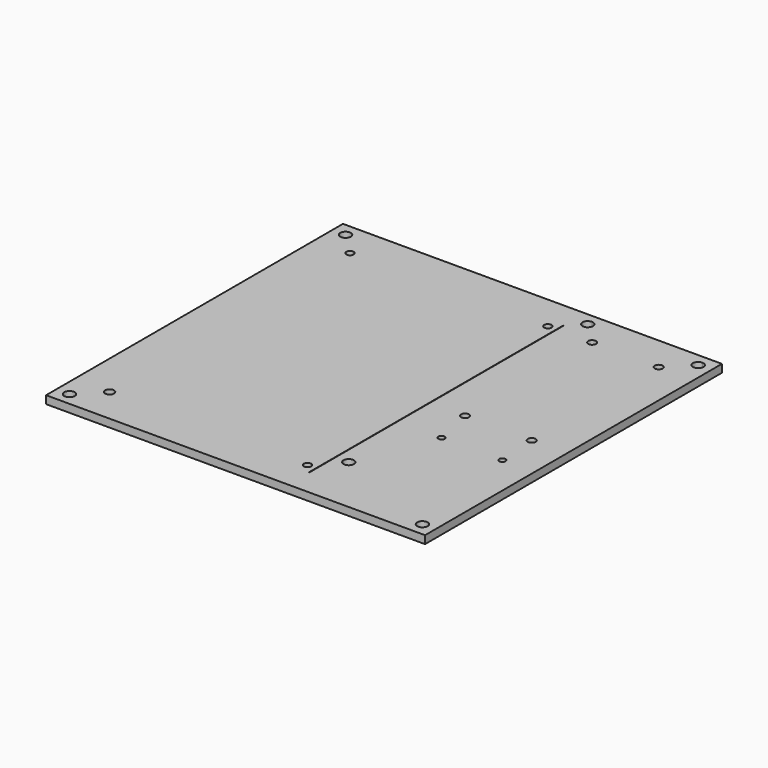
from build123d import *

# Parameters (mm, degrees)
F0_R     = 1.5
F0_W     = 3
F0_H     = 5
F0_W_2   = 4
F0_H_2   = 75.28
F0_H_3   = 40.64
F0_H_4   = 5.08
F1_DEPTH = 3


# Not quite as in the source:
# - a feature names something its author has since deleted; it is built from what else it names


with BuildPart() as f1:
    # F0 (on Top) → F1 (new body)
    with BuildSketch(Plane.XY):
        with BuildLine():
            Line((-134.3440142274, -1.256315279), (-139.3440142274, -1.256315279))
            Line((-139.3440142274, -1.256315279), (-139.3440142274, -6.256315279))
            Line((-139.3440142274, -6.256315279), (-136.3440142274, -6.256315279))
            ThreePointArc((-136.3440142274, -6.256315279), (-135.7582277898, -4.8421017166), (-134.3440142274, -4.256315279))
            Line((-134.3440142274, -4.256315279), (-134.3440142274, -1.256315279))
        make_face()
        Polygon((-139.3440142274, -6.256315279), (-139.3440142274, -1.256315279), (-221.3440142274, -1.256315279), (-221.3440142274, -6.256315279), (-221.3440142274, -11.256315279), (-217.9440142274, -11.256315279), (-151.4240142274, -11.256315279), (-147.4240142274, -11.256315279), (-142.7440142274, -11.256315279), (-139.4949736476, -11.256315279), (-139.3440142274, -11.256315279), align=None)
        with BuildLine():
            Line((-129.3440142274, -1.256315279), (-134.3440142274, -1.256315279))
            Line((-134.3440142274, -1.256315279), (-134.3440142274, -4.256315279))
            ThreePointArc((-134.3440142274, -4.256315279), (-132.929800665, -4.8421017166), (-132.3440142274, -6.256315279))
            ThreePointArc((-132.3440142274, -6.256315279), (-134.3440142274, -8.256315279), (-136.3440142274, -6.256315279))
            Line((-136.3440142274, -6.256315279), (-139.3440142274, -6.256315279))
            Line((-139.3440142274, -6.256315279), (-139.3440142274, -11.256315279))
            Line((-139.3440142274, -11.256315279), (-129.3440142274, -11.256315279))
            Line((-129.3440142274, -11.256315279), (-129.3440142274, -6.256315279))
            Line((-129.3440142274, -6.256315279), (-129.3440142274, -1.256315279))
        make_face()
        with BuildLine():
            Line((-221.3440142274, -6.256315279), (-221.3440142274, -1.256315279))
            Line((-221.3440142274, -1.256315279), (-231.3440142274, -1.256315279))
            Line((-231.3440142274, -1.256315279), (-231.3440142274, -132.256315279))
            Line((-231.3440142274, -132.256315279), (-221.3440142274, -132.256315279))
            Line((-221.3440142274, -132.256315279), (-221.3440142274, -128.856315279))
            Line((-221.3440142274, -128.856315279), (-221.3440142274, -14.656315279))
            Line((-221.3440142274, -14.656315279), (-221.3440142274, -11.256315279))
            Line((-221.3440142274, -11.256315279), (-226.3440142274, -11.256315279))
            Line((-226.3440142274, -11.256315279), (-226.3440142274, -8.256315279))
            ThreePointArc((-226.3440142274, -8.256315279), (-227.7582277898, -4.8421017166), (-224.3440142274, -6.256315279))
            Line((-224.3440142274, -6.256315279), (-221.3440142274, -6.256315279))
        make_face()
        with BuildLine():
            Line((-92.3440142274, -1.256315279), (-129.3440142274, -1.256315279))
            Line((-129.3440142274, -1.256315279), (-129.3440142274, -6.256315279))
            Line((-129.3440142274, -6.256315279), (-126.3440142274, -6.256315279))
            Line((-126.3440142274, -6.256315279), (-100.3440142274, -6.256315279))
            Line((-100.3440142274, -6.256315279), (-97.3440142274, -6.256315279))
            Line((-97.3440142274, -6.256315279), (-97.3440142274, -11.256315279))
            Line((-97.3440142274, -11.256315279), (-97.3440142274, -14.596315279))
            Line((-97.3440142274, -14.596315279), (-97.3440142274, -74.916315279))
            Line((-97.3440142274, -74.916315279), (-97.3440142274, -78.256315279))
            Line((-97.3440142274, -78.256315279), (-100.6840142274, -78.256315279))
            Line((-100.6840142274, -78.256315279), (-126.0040142274, -78.256315279))
            Line((-126.0040142274, -78.256315279), (-129.3440142274, -78.256315279))
            Line((-129.3440142274, -78.256315279), (-129.3440142274, -108.756315279))
            Line((-129.3440142274, -108.756315279), (-129.3440142274, -111.756315279))
            Line((-129.3440142274, -111.756315279), (-129.3440142274, -114.756315279))
            Line((-129.3440142274, -114.756315279), (-129.3440142274, -124.756315279))
            Line((-129.3440142274, -124.756315279), (-129.3440142274, -142.256315279))
            Line((-129.3440142274, -142.256315279), (-92.3440142274, -142.256315279))
            Line((-92.3440142274, -142.256315279), (-92.3440142274, -139.256315279))
            ThreePointArc((-92.3440142274, -139.256315279), (-93.7582277898, -135.8421017166), (-90.3440142274, -137.256315279))
            Line((-90.3440142274, -137.256315279), (-87.3440142274, -137.256315279))
            Line((-87.3440142274, -137.256315279), (-87.3440142274, -6.256315279))
            Line((-87.3440142274, -6.256315279), (-90.3440142274, -6.256315279))
            ThreePointArc((-90.3440142274, -6.256315279), (-93.7582277898, -7.6705288414), (-92.3440142274, -4.256315279))
            Line((-92.3440142274, -4.256315279), (-92.3440142274, -1.256315279))
        make_face()
        Polygon((-97.8440142274, -124.5755243927), (-124.3440142274, -124.5755243927), (-124.3440142274, -90.2755243927), (-124.3440142274, -88.5755243927), (-122.6440142274, -88.5755243927), (-99.5440142274, -88.5755243927), (-97.8440142274, -88.5755243927), (-97.8440142274, -90.2755243927), align=None, mode=Mode.SUBTRACT)
        Polygon((-129.3440142274, -11.256315279), (-139.3440142274, -11.256315279), (-139.3440142274, -14.656315279), (-139.3440142274, -114.756315279), (-129.3440142274, -114.756315279), (-129.3440142274, -111.756315279), (-129.3440142274, -108.756315279), (-129.3440142274, -78.256315279), (-129.3440142274, -74.916315279), (-129.3440142274, -27.956315279), (-129.3440142274, -27.456315279), (-129.3440142274, -14.596315279), (-129.3440142274, -14.056315279), align=None)
        with BuildLine():
            Line((-221.3440142274, -11.256315279), (-221.3440142274, -6.256315279))
            Line((-221.3440142274, -6.256315279), (-224.3440142274, -6.256315279))
            ThreePointArc((-224.3440142274, -6.256315279), (-224.929800665, -7.6705288414), (-226.3440142274, -8.256315279))
            Line((-226.3440142274, -8.256315279), (-226.3440142274, -11.256315279))
            Line((-226.3440142274, -11.256315279), (-221.3440142274, -11.256315279))
        make_face()
        Polygon((-126.3440142274, -6.256315279), (-129.3440142274, -6.256315279), (-129.3440142274, -11.256315279), (-126.5440142274, -11.256315279), (-126.3440142274, -11.256315279), align=None)
        with BuildLine():
            Line((-87.3440142274, -1.256315279), (-92.3440142274, -1.256315279))
            Line((-92.3440142274, -1.256315279), (-92.3440142274, -4.256315279))
            ThreePointArc((-92.3440142274, -4.256315279), (-90.929800665, -4.8421017166), (-90.3440142274, -6.256315279))
            Line((-90.3440142274, -6.256315279), (-87.3440142274, -6.256315279))
            Line((-87.3440142274, -6.256315279), (-87.3440142274, -1.256315279))
        make_face()
        Polygon((-126.5440142274, -11.256315279), (-129.3440142274, -11.256315279), (-129.3440142274, -14.056315279), (-129.3440142274, -14.596315279), (-129.3440142274, -27.456315279), (-129.3440142274, -27.956315279), (-129.3440142274, -74.916315279), (-129.3440142274, -78.256315279), (-126.0040142274, -78.256315279), (-100.6840142274, -78.256315279), (-97.3440142274, -78.256315279), (-97.3440142274, -74.916315279), (-97.3440142274, -14.596315279), (-97.3440142274, -11.256315279), (-100.3440142274, -11.256315279), (-100.6840142274, -11.256315279), (-126.0040142274, -11.256315279), (-126.3440142274, -11.256315279), align=None)
        with Locations((-126.0040142274, -74.916315279)):
            Circle(F0_R, mode=Mode.SUBTRACT)
        with Locations((-100.6840142274, -74.916315279)):
            Circle(F0_R, mode=Mode.SUBTRACT)
        with Locations((-126.0040142274, -14.596315279)):
            Circle(F0_R, mode=Mode.SUBTRACT)
        with Locations((-100.6840142274, -14.596315279)):
            Circle(F0_R, mode=Mode.SUBTRACT)
        with BuildLine():
            Line((-139.4949736476, -14.656315279), (-139.4949736476, -11.256315279))
            Line((-139.4949736476, -11.256315279), (-142.7440142274, -11.256315279))
            Line((-142.7440142274, -11.256315279), (-142.7440142274, -13.256315279))
            ThreePointArc((-142.7440142274, -13.256315279), (-141.7540647337, -13.6663657853), (-141.3440142274, -14.656315279))
            Line((-141.3440142274, -14.656315279), (-139.4949736476, -14.656315279))
        make_face()
        with BuildLine():
            Line((-217.9440142274, -11.256315279), (-221.3440142274, -11.256315279))
            Line((-221.3440142274, -11.256315279), (-221.3440142274, -14.656315279))
            Line((-221.3440142274, -14.656315279), (-219.3440142274, -14.656315279))
            ThreePointArc((-219.3440142274, -14.656315279), (-218.9339637211, -13.6663657853), (-217.9440142274, -13.256315279))
            Line((-217.9440142274, -13.256315279), (-217.9440142274, -11.256315279))
        make_face()
        with BuildLine():
            Line((-221.3440142274, -132.256315279), (-231.3440142274, -132.256315279))
            Line((-231.3440142274, -132.256315279), (-231.3440142274, -137.3912245035))
            Line((-231.3440142274, -137.3912245035), (-228.3440142274, -137.3912245035))
            ThreePointArc((-228.3440142274, -137.3912245035), (-226.3440142274, -135.3912245035), (-224.3440142274, -137.3912245035))
            ThreePointArc((-224.3440142274, -137.3912245035), (-224.929800665, -138.8054380659), (-226.3440142274, -139.3912245035))
            Line((-226.3440142274, -139.3912245035), (-226.3440142274, -142.256315279))
            Line((-226.3440142274, -142.256315279), (-221.3440142274, -142.256315279))
            Line((-221.3440142274, -142.256315279), (-221.3440142274, -132.256315279))
        make_face()
        Polygon((-100.3440142274, -6.256315279), (-126.3440142274, -6.256315279), (-126.3440142274, -11.256315279), (-126.0040142274, -11.256315279), (-100.6840142274, -11.256315279), (-100.3440142274, -11.256315279), align=None)
        with BuildLine():
            Line((-139.4949736476, -128.856315279), (-139.4949736476, -14.656315279))
            Line((-139.4949736476, -14.656315279), (-141.3440142274, -14.656315279))
            ThreePointArc((-141.3440142274, -14.656315279), (-143.7339637211, -15.6462647727), (-142.7440142274, -13.256315279))
            Line((-142.7440142274, -13.256315279), (-142.7440142274, -11.256315279))
            Line((-142.7440142274, -11.256315279), (-147.4240142274, -11.256315279))
            Line((-147.4240142274, -11.256315279), (-147.4240142274, -86.536315279))
            Line((-147.4240142274, -86.536315279), (-147.4240142274, -127.176315279))
            Line((-147.4240142274, -127.176315279), (-147.4240142274, -132.256315279))
            Line((-147.4240142274, -132.256315279), (-142.7440142274, -132.256315279))
            Line((-142.7440142274, -132.256315279), (-142.7440142274, -130.256315279))
            ThreePointArc((-142.7440142274, -130.256315279), (-143.7339637211, -127.8663657853), (-141.3440142274, -128.856315279))
            Line((-141.3440142274, -128.856315279), (-139.4949736476, -128.856315279))
        make_face()
        with BuildLine():
            Line((-129.3440142274, -114.756315279), (-139.3440142274, -114.756315279))
            Line((-139.3440142274, -114.756315279), (-139.3440142274, -119.756315279))
            Line((-139.3440142274, -119.756315279), (-136.3440142274, -119.756315279))
            ThreePointArc((-136.3440142274, -119.756315279), (-134.3440142274, -117.756315279), (-132.3440142274, -119.756315279))
            ThreePointArc((-132.3440142274, -119.756315279), (-132.929800665, -121.1705288414), (-134.3440142274, -121.756315279))
            Line((-134.3440142274, -121.756315279), (-134.3440142274, -124.756315279))
            Line((-134.3440142274, -124.756315279), (-129.3440142274, -124.756315279))
            Line((-129.3440142274, -124.756315279), (-129.3440142274, -114.756315279))
        make_face()
        with BuildLine():
            Line((-151.4240142274, -11.256315279), (-217.9440142274, -11.256315279))
            Line((-217.9440142274, -11.256315279), (-217.9440142274, -13.256315279))
            ThreePointArc((-217.9440142274, -13.256315279), (-216.9540647337, -13.6663657853), (-216.5440142274, -14.656315279))
            ThreePointArc((-216.5440142274, -14.656315279), (-217.9440142274, -16.056315279), (-219.3440142274, -14.656315279))
            Line((-219.3440142274, -14.656315279), (-221.3440142274, -14.656315279))
            Line((-221.3440142274, -14.656315279), (-221.3440142274, -128.856315279))
            Line((-221.3440142274, -128.856315279), (-219.6440142274, -128.856315279))
            ThreePointArc((-219.6440142274, -128.856315279), (-217.9440142274, -127.156315279), (-216.2440142274, -128.856315279))
            ThreePointArc((-216.2440142274, -128.856315279), (-216.7419326994, -130.058396807), (-217.9440142274, -130.556315279))
            Line((-217.9440142274, -130.556315279), (-217.9440142274, -132.256315279))
            Line((-217.9440142274, -132.256315279), (-151.4240142274, -132.256315279))
            Line((-151.4240142274, -132.256315279), (-151.4240142274, -127.176315279))
            Line((-151.4240142274, -127.176315279), (-151.4240142274, -86.536315279))
            Line((-151.4240142274, -86.536315279), (-151.4240142274, -11.256315279))
        make_face()
        with BuildLine():
            Line((-221.3440142274, -128.856315279), (-221.3440142274, -132.256315279))
            Line((-221.3440142274, -132.256315279), (-217.9440142274, -132.256315279))
            Line((-217.9440142274, -132.256315279), (-217.9440142274, -130.556315279))
            ThreePointArc((-217.9440142274, -130.556315279), (-219.1460957554, -130.058396807), (-219.6440142274, -128.856315279))
            Line((-219.6440142274, -128.856315279), (-221.3440142274, -128.856315279))
        make_face()
        Polygon((-217.9440142274, -132.256315279), (-221.3440142274, -132.256315279), (-221.3440142274, -142.256315279), (-139.3440142274, -142.256315279), (-139.4949736476, -132.256315279), (-142.7440142274, -132.256315279), (-147.4240142274, -132.256315279), (-151.4240142274, -132.256315279), align=None)
        with BuildLine():
            Line((-228.3440142274, -137.3912245035), (-231.3440142274, -137.3912245035))
            Line((-231.3440142274, -137.3912245035), (-231.3440142274, -142.256315279))
            Line((-231.3440142274, -142.256315279), (-226.3440142274, -142.256315279))
            Line((-226.3440142274, -142.256315279), (-226.3440142274, -139.3912245035))
            ThreePointArc((-226.3440142274, -139.3912245035), (-227.7582277898, -138.8054380659), (-228.3440142274, -137.3912245035))
        make_face()
        with Locations((-98.8440142274, -8.756315279)):
            Rectangle(F0_W, F0_H)
        with BuildLine():
            Line((-139.4949736476, -132.256315279), (-139.4949736476, -128.856315279))
            Line((-139.4949736476, -128.856315279), (-141.3440142274, -128.856315279))
            ThreePointArc((-141.3440142274, -128.856315279), (-141.7540647337, -129.8462647727), (-142.7440142274, -130.256315279))
            Line((-142.7440142274, -130.256315279), (-142.7440142274, -132.256315279))
            Line((-142.7440142274, -132.256315279), (-139.4949736476, -132.256315279))
        make_face()
        with Locations((-149.4240142274, -48.896315279)):
            Rectangle(F0_W_2, F0_H_2)
        with BuildLine():
            Line((-136.3440142274, -119.756315279), (-139.3440142274, -119.756315279))
            Line((-139.3440142274, -119.756315279), (-139.3440142274, -124.756315279))
            Line((-139.3440142274, -124.756315279), (-139.1930548072, -124.756315279))
            Line((-139.1930548072, -124.756315279), (-134.3440142274, -124.756315279))
            Line((-134.3440142274, -124.756315279), (-134.3440142274, -121.756315279))
            ThreePointArc((-134.3440142274, -121.756315279), (-135.7582277898, -121.1705288414), (-136.3440142274, -119.756315279))
        make_face()
        with BuildLine():
            Line((-87.3440142274, -142.256315279), (-87.3440142274, -137.256315279))
            Line((-87.3440142274, -137.256315279), (-90.3440142274, -137.256315279))
            ThreePointArc((-90.3440142274, -137.256315279), (-90.929800665, -138.6705288414), (-92.3440142274, -139.256315279))
            Line((-92.3440142274, -139.256315279), (-92.3440142274, -142.256315279))
            Line((-92.3440142274, -142.256315279), (-87.3440142274, -142.256315279))
        make_face()
        Polygon((-139.3440142274, -132.256315279), (-139.4949736476, -132.256315279), (-139.3440142274, -142.256315279), (-129.3440142274, -142.256315279), (-129.3440142274, -124.756315279), (-134.3440142274, -124.756315279), (-139.1930548072, -124.756315279), (-139.3440142274, -124.756315279), (-139.3440142274, -128.856315279), align=None)
        with Locations((-149.4240142274, -106.856315279)):
            Rectangle(F0_W_2, F0_H_3)
        with Locations((-149.4240142274, -129.716315279)):
            Rectangle(F0_W_2, F0_H_4)
        with BuildLine():
            Line((-124.3440142274, -90.2755243927), (-124.3440142274, -124.5755243927))
            Line((-124.3440142274, -124.5755243927), (-97.8440142274, -124.5755243927))
            Line((-97.8440142274, -124.5755243927), (-97.8440142274, -90.2755243927))
            Line((-97.8440142274, -90.2755243927), (-98.3440142274, -90.2755243927))
            ThreePointArc((-98.3440142274, -90.2755243927), (-100.3925423648, -91.1240525301), (-99.5440142274, -89.0755243927))
            Line((-99.5440142274, -89.0755243927), (-99.5440142274, -88.5755243927))
            Line((-99.5440142274, -88.5755243927), (-122.6440142274, -88.5755243927))
            Line((-122.6440142274, -88.5755243927), (-122.6440142274, -89.0755243927))
            ThreePointArc((-122.6440142274, -89.0755243927), (-121.79548609, -89.4269962553), (-121.4440142274, -90.2755243927))
            ThreePointArc((-121.4440142274, -90.2755243927), (-122.6440142274, -91.4755243927), (-123.8440142274, -90.2755243927))
            Line((-123.8440142274, -90.2755243927), (-124.3440142274, -90.2755243927))
        make_face()
        with BuildLine():
            Line((-124.3440142274, -88.5755243927), (-124.3440142274, -90.2755243927))
            Line((-124.3440142274, -90.2755243927), (-123.8440142274, -90.2755243927))
            ThreePointArc((-123.8440142274, -90.2755243927), (-123.4925423648, -89.4269962553), (-122.6440142274, -89.0755243927))
            Line((-122.6440142274, -89.0755243927), (-122.6440142274, -88.5755243927))
            Line((-122.6440142274, -88.5755243927), (-124.3440142274, -88.5755243927))
        make_face()
        with BuildLine():
            Line((-98.3440142274, -90.2755243927), (-97.8440142274, -90.2755243927))
            Line((-97.8440142274, -90.2755243927), (-97.8440142274, -88.5755243927))
            Line((-97.8440142274, -88.5755243927), (-99.5440142274, -88.5755243927))
            Line((-99.5440142274, -88.5755243927), (-99.5440142274, -89.0755243927))
            ThreePointArc((-99.5440142274, -89.0755243927), (-98.69548609, -89.4269962553), (-98.3440142274, -90.2755243927))
        make_face()
    extrude(amount=F1_DEPTH)


solid = f1.part
